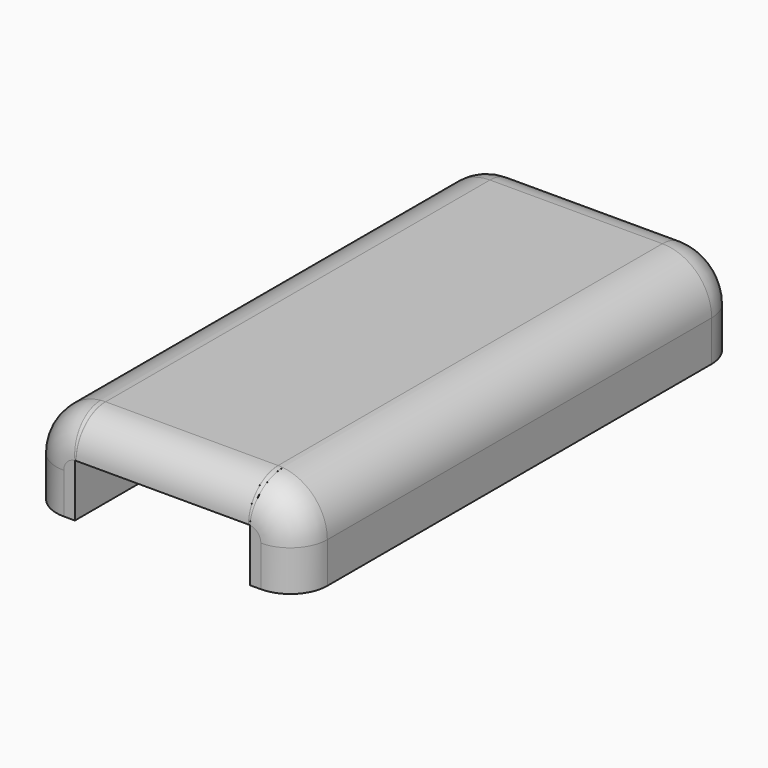
from build123d import *

# Parameters (mm, degrees)
F1_DEPTH  = 45
F3_W      = 4
F3_H      = 4.3
F4_DEPTH  = 16
F6_D      = 4.5
F6_DEPTH  = 30
F6_TIP    = 1.3519363928
F8_R      = 4
F11_W     = 8
F11_H     = 4.3
F12_DEPTH = 0.9
F13_W     = 8
F13_H     = 4.3
F14_DEPTH = 0.9
F15_R     = 2.99999
F2_R      = 1.95
F2_R_2    = 0.75
F16_DEPTH = 4.3


# Not quite as in the source:
# - a fillet or chamfer is up to 0.001 mm smaller than in the source, because OpenCascade refuses the exact size


with BuildPart() as f1:
    # F0 (on Front) → F1 (new body)
    with BuildSketch(Plane.XZ):
        Polygon((0, 0), (0, 4.3), (16, 4.3), (16, 0), (19, 0), (19, 7.3), (-3, 7.3), (-3, 0), align=None)
    extrude(amount=F1_DEPTH)

    # F3 (on face) → F4 (join)
    with BuildSketch(Plane.YZ):
        with Locations((-2, 2.15)):
            Rectangle(F3_W, F3_H)
    extrude(amount=F4_DEPTH)

    # F6
    with Locations(Plane(origin=(0, 0, 0), x_dir=(-1, 0, 0), z_dir=(0, 1, 0))):
        with Locations((-8, 0)):
            Hole(F6_D / 2, depth=F6_DEPTH)
            with Locations((0, 0, -(F6_DEPTH + F6_TIP / 2))):  # 118° drill point
                Cone(0, F6_D / 2, F6_TIP, mode=Mode.SUBTRACT)


with BuildPart() as f7_1:
    # F7: copy of F1
    add(f1.part.moved(Location((31.9, 0.1, 0))))


with BuildPart() as f1_1:
    add(f1.part)

    # F8
    f8_edges = [f1_1.edges().sort_by_distance(p)[0] for p in [
        (-3, -22.5, 7.3),
        (19, -22.5, 7.3),
    ]]
    fillet(f8_edges, radius=F8_R)


with BuildPart() as f10_1:
    # F10: copy of F1
    add(f1_1.part.moved(Location((35.6, 1.7, 0))))


with BuildPart() as f1_2:
    add(f1_1.part)

    # F11 (on face) → F12 (join)
    with BuildSketch(Plane.YZ):
        with Locations((-41, 2.15)):
            Rectangle(F11_W, F11_H)
    extrude(amount=F12_DEPTH)

    # F13 (on face) → F14 (join)
    with BuildSketch(Plane(origin=(16, 0, 0), x_dir=(0, -1, 0), z_dir=(-1, 0, 0))):
        with Locations((41, 2.15)):
            Rectangle(F13_W, F13_H)
    extrude(amount=F14_DEPTH)

    # F15 (radius 3 in the source; OpenCascade refuses exactly that, so slightly less here)
    f15_edges = [f1_2.edges().sort_by_distance(p)[0] for p in [
        (8, -45, 7.3),
        (8, 0, 7.3),
    ]]
    fillet(f15_edges, radius=F15_R)

    # F2 (on face) → F16 (join)
    with BuildSketch(Plane(origin=(0, 0, 4.3), x_dir=(1, 0, 0), z_dir=(0, 0, -1))):
        with Locations((2, 30)):
            Circle(F2_R)
        with Locations((2, 30)):
            Circle(F2_R_2, mode=Mode.SUBTRACT)
        with Locations((14, 30)):
            Circle(F2_R)
        with Locations((14, 30)):
            Circle(F2_R_2, mode=Mode.SUBTRACT)
        with Locations((2, 8)):
            Circle(F2_R)
        with Locations((2, 8)):
            Circle(F2_R_2, mode=Mode.SUBTRACT)
        with Locations((14, 8)):
            Circle(F2_R)
        with Locations((14, 8)):
            Circle(F2_R_2, mode=Mode.SUBTRACT)
    extrude(amount=F16_DEPTH)


solid = f1_2.part
